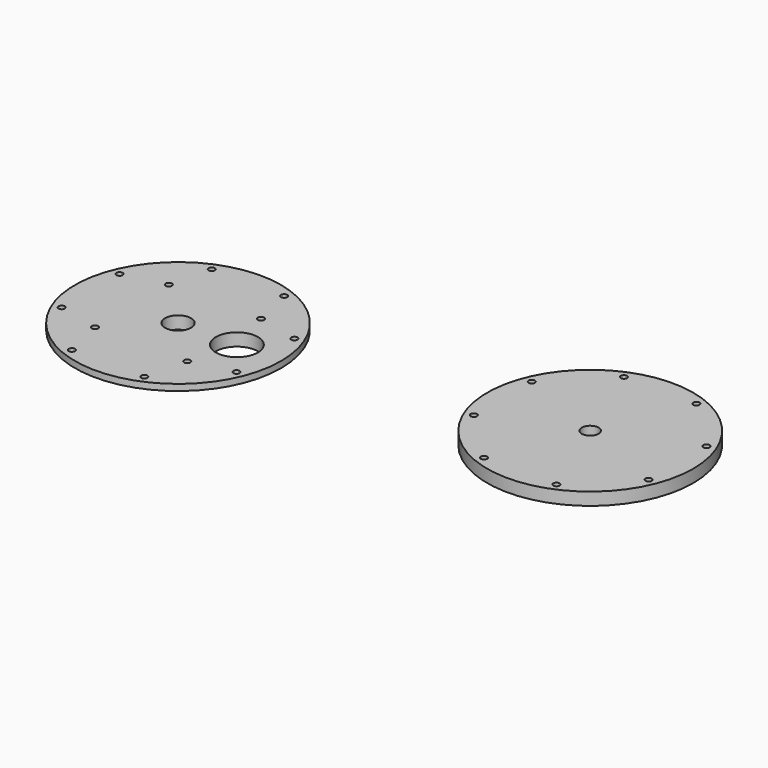
from build123d import *

# Parameters (mm, degrees)
F0_R      = 155.575
F0_R_2    = 126.365
F0_R_3    = 19.685
F1_DEPTH  = 19.05
F2_DEPTH  = 9.525
F3_R      = 4.7625
F4_DEPTH  = 25.4
F8_R      = 155.575
F8_R_2    = 12.7
F9_DEPTH  = 19.05
F10_R     = 4.7625
F11_DEPTH = 25.4
F12_R     = 31.75
F13_DEPTH = 50.8
F14_R     = 4.7625
F15_DEPTH = 12.7
F17_R     = 127
F17_R_2   = 124.7775
F18_DEPTH = 3.175
F19_SIZE  = 0.254


with BuildPart() as f1:
    # F0 (on Top) → F1 (new body)
    with BuildSketch(Plane.XY):
        Circle(F0_R)
        Circle(F0_R_2, mode=Mode.SUBTRACT)
        Circle(F0_R_2)
        Circle(F0_R_3, mode=Mode.SUBTRACT)
    extrude(amount=F1_DEPTH)

    # F0 (on Top) → F2 (cut)
    with BuildSketch(Plane.XY):
        Circle(F0_R)
        Circle(F0_R_2, mode=Mode.SUBTRACT)
    extrude(amount=F2_DEPTH, mode=Mode.SUBTRACT)

    # F3 (on face) → F4 (cut)
    with BuildSketch(Plane.XY.offset(19.05)):
        with Locations((-54.6758953992, 131.9992882076)):
            Circle(F3_R)
        with Locations((-131.9992882076, 54.6758953992)):
            Circle(F3_R)
        with Locations((-131.9992882076, -54.6758953992)):
            Circle(F3_R)
        with Locations((-54.6758953992, -131.9992882076)):
            Circle(F3_R)
        with Locations((54.6758953992, -131.9992882076)):
            Circle(F3_R)
        with Locations((131.9992882076, -54.6758953992)):
            Circle(F3_R)
        with Locations((131.9992882076, 54.6758953992)):
            Circle(F3_R)
        with Locations((54.6758953992, 131.9992882076)):
            Circle(F3_R)
    extrude(amount=-F4_DEPTH, mode=Mode.SUBTRACT)

    # F12 (on face) → F13 (cut)
    with BuildSketch(Plane.XY.offset(19.05)):
        with Locations((88.9, 0)):
            Circle(F12_R)
    extrude(amount=-F13_DEPTH, mode=Mode.SUBTRACT)

    # F14 (on face) → F15 (cut)
    with BuildSketch(Plane.XY.offset(19.05)):
        with Locations((-69.5969849383, 69.5969849383)):
            Circle(F14_R)
        with Locations((-69.5969849383, -69.5969849383)):
            Circle(F14_R)
        with Locations((69.5969849383, -69.5969849383)):
            Circle(F14_R)
        with Locations((69.5969849383, 69.5969849383)):
            Circle(F14_R)
    extrude(amount=-F15_DEPTH, mode=Mode.SUBTRACT)

    # F17 (on offset) → F18 (cut)
    with BuildSketch(Plane(origin=(0, 0, 3.175), x_dir=(1, 0, 0), z_dir=(0, 0, -1))):
        Circle(F17_R)
        Circle(F17_R_2, mode=Mode.SUBTRACT)
    extrude(amount=-F18_DEPTH, mode=Mode.SUBTRACT)

    # F19
    f19_edges = [f1.edges().sort_by_distance(p)[0] for p in [
        (-126.365, 0, 6.35),
        (-126.365, 0, 3.175),
    ]]
    chamfer(f19_edges, length=F19_SIZE)


with BuildPart() as f9:
    # F8 (on offset) → F9 (new body)
    with BuildSketch(Plane(origin=(0, 0, 6.35), x_dir=(1, 0, 0), z_dir=(0, 0, -1))):
        with Locations((536.0572338104, -107.8919991851)):
            Circle(F8_R)
        with Locations((536.0572338104, -107.8919991851)):
            Circle(F8_R_2, mode=Mode.SUBTRACT)
    extrude(amount=F9_DEPTH)

    # F10 (on face) → F11 (cut)
    with BuildSketch(Plane.XY.offset(6.35)):
        with Locations((481.3813384113, 239.8912873926)):
            Circle(F10_R)
        with Locations((404.0579456029, 162.5678945842)):
            Circle(F10_R)
        with Locations((404.0579456029, 53.2161037859)):
            Circle(F10_R)
        with Locations((481.3813384113, -24.1072890225)):
            Circle(F10_R)
        with Locations((590.7331292096, -24.1072890225)):
            Circle(F10_R)
        with Locations((668.056522018, 53.2161037859)):
            Circle(F10_R)
        with Locations((668.056522018, 162.5678945842)):
            Circle(F10_R)
        with Locations((590.7331292096, 239.8912873926)):
            Circle(F10_R)
    extrude(amount=-F11_DEPTH, mode=Mode.SUBTRACT)


solid = Compound([f1.part, f9.part])
